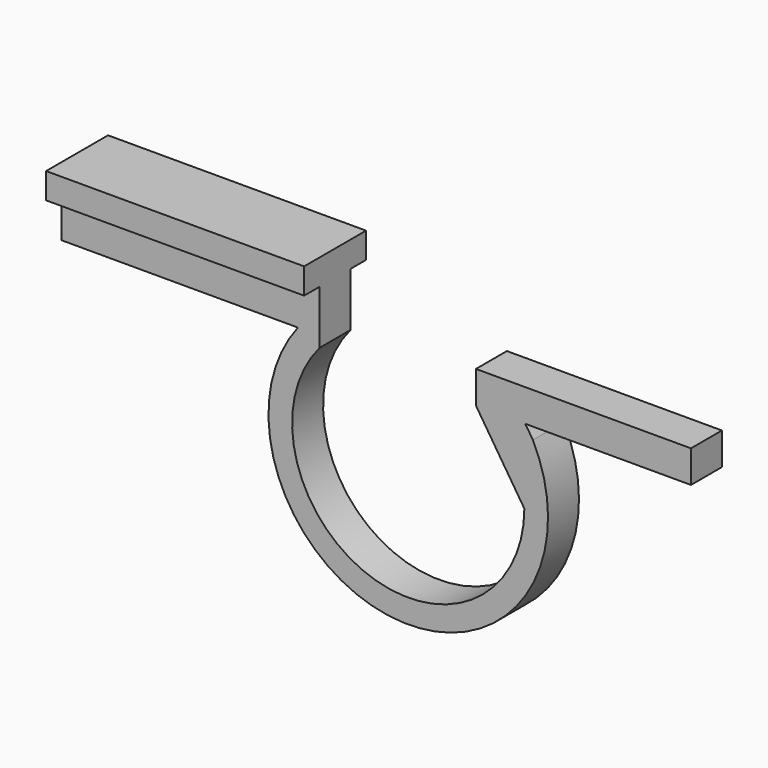
from build123d import *

# Parameters (mm, degrees)
F1_DEPTH = 1.143
F2_DEPTH = 1.143
F4_DEPTH = 15.24


# Not quite as in the source:
# - a feature names something its author has since deleted; it is built from what else it names


with BuildPart() as f1:
    # F0 (on Front) → F1 (new body, symmetric)
    with BuildSketch(Plane.XZ):
        with BuildLine():
            Line((0, 1.905), (0, 0))
            Line((0, 0), (2.8609845606, -4.4301707429))
            ThreePointArc((2.8609845606, -4.4301707429), (-6.3560607273, -10.8696636833), (-9.232065696, 0))
            Line((-9.232065696, 0), (-9.232065696, 0.635))
            Line((-9.232065696, 0.635), (-10.5153795245, 0.635))
            ThreePointArc((-10.5153795245, 0.635), (-4.785192357, -12.6474575303), (3.3653166944, -0.6963937609))
            Line((3.3653166944, -0.6963937609), (2.9155887012, 0))
            Line((2.9155887012, 0), (12.7, 0))
            Line((12.7, 0), (12.7, 1.905))
            Line((12.7, 1.905), (0, 1.905))
        make_face()
    extrude(amount=F1_DEPTH, both=True)

    # F0 (on Front) → F2 (join, symmetric)
    with BuildSketch(Plane.XZ):
        Polygon((-10.5153795245, 0.635), (-9.232065696, 0.635), (-9.232065696, 3.175), (-24.472065696, 3.175), (-24.472065696, 0.635), align=None)
    extrude(amount=F2_DEPTH, both=True)

    # F3 (on face) → F4 (join, through all)
    with BuildSketch(Plane(origin=(-24.472065696, 0, 0), x_dir=(0, -1, 0), z_dir=(-1, 0, 0))):
        Polygon((-2.286, 4.699), (-2.286, 3.175), (0, 3.175), (2.286, 3.175), (2.286, 4.699), (0, 4.699), align=None)
    extrude(amount=-F4_DEPTH)


solid = f1.part
